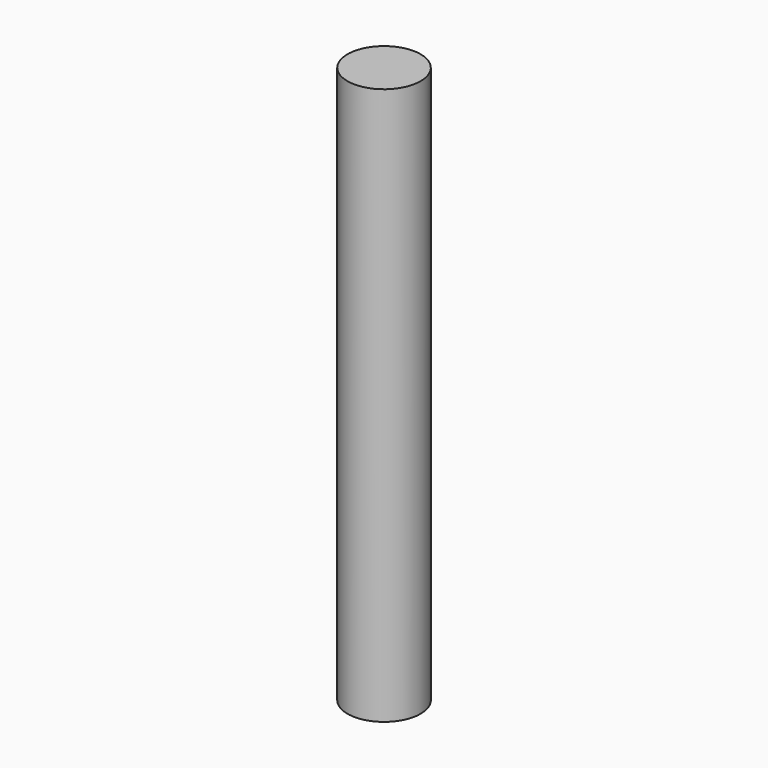
from build123d import *

# Parameters (mm, degrees)
F0_R     = 1.25
F1_DEPTH = 19.05


# Not quite as in the source:
# - a length typed as a fraction of an inch, garbled in the dataset ("3 / 203.2 mm" for 3/8 in), is restored


with BuildPart() as f1:
    # F0 (on Top) → F1 (new body)
    with BuildSketch(Plane.XY):
        with Locations((-41.4591245353, 15.7053414732)):
            Circle(F0_R)
    extrude(amount=F1_DEPTH)


solid = f1.part
